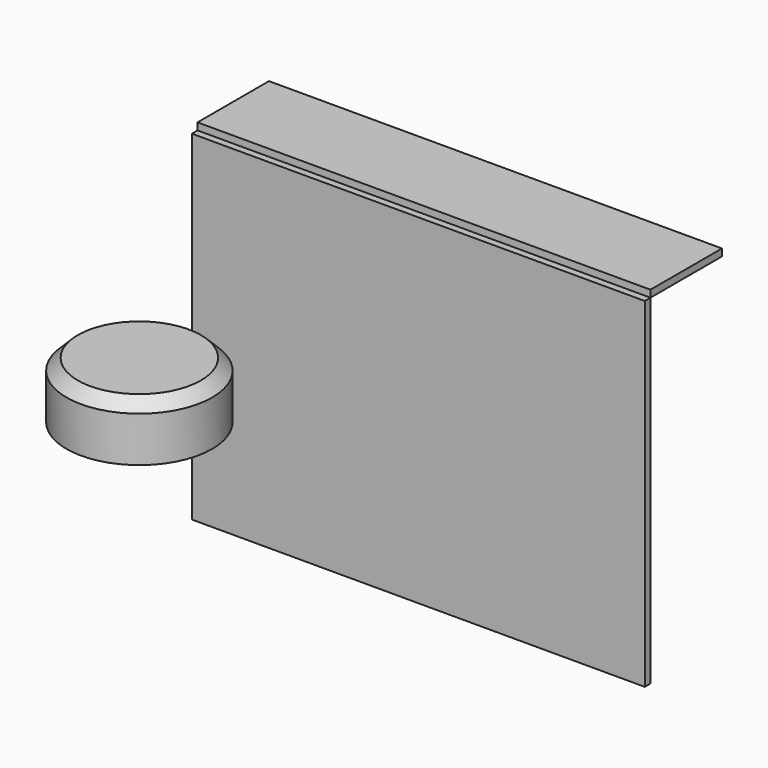
from build123d import *

# Parameters (mm, degrees)
F0_W     = 203.2
F0_H     = 152.4
F1_DEPTH = 3.175
F2_W     = 203.2
F2_H     = 40.0667153299
F3_DEPTH = 3.175
F5_R     = 32.6737940356
F6_DEPTH = 25.4
F8_SIZE  = 5.08


# Not quite as in the source:
# - the program builds the solid bodies; features that only make, move or delete a surface that nothing else refers to are left out


with BuildPart() as f1:
    # F0 (on Front) → F1 (new body)
    with BuildSketch(Plane.XZ):
        Rectangle(F0_W, F0_H)
    extrude(amount=F1_DEPTH)


with BuildPart() as f3:
    # F2 (on face) → F3 (new body)
    with BuildSketch(Plane.XY.offset(76.2)):
        with Locations((0, 20.0333576649)):
            Rectangle(F2_W, F2_H)
    extrude(amount=F3_DEPTH)


with BuildPart() as f6:
    # F5 (on Top) → F6 (new body)
    with BuildSketch(Plane.XY):
        with Locations((-70.7184076309, -71.2099298835)):
            Circle(F5_R)
    extrude(amount=F6_DEPTH)

    # F8
    f8_edges = [f6.edges().sort_by_distance(p)[0] for p in [
        (-103.392202, -71.20993, 25.4),
    ]]
    chamfer(f8_edges, length=F8_SIZE)


solid = Compound([f1.part, f3.part, f6.part])
